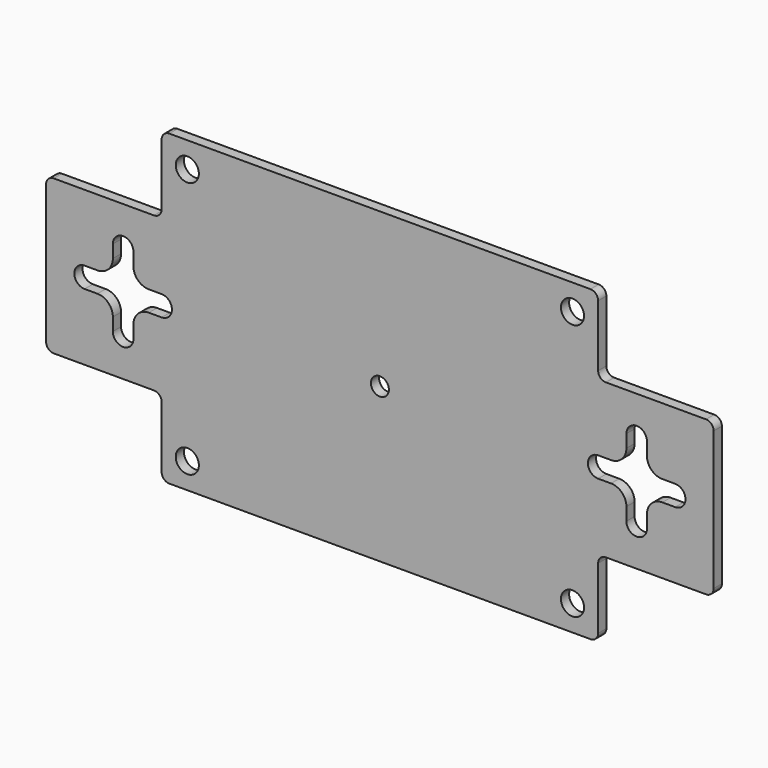
from build123d import *

# Parameters (mm, degrees)
F0_W     = 85
F0_H     = 15
F0_R     = 2.25
F0_R_2   = 1.75
F1_DEPTH = 2
F2_R     = 1.5
F3_R     = 3


# Not quite as in the source:
# - a feature names something its author has since deleted; it is built from what else it names


with BuildPart() as f1:
    # F0 (on Front) → F1 (new body)
    with BuildSketch(Plane.XZ):
        with Locations((0, 22.5)):
            Rectangle(F0_W, F0_H)
        with Locations((-37.5, 25)):
            Circle(F0_R, mode=Mode.SUBTRACT)
        with Locations((37.5, 25)):
            Circle(F0_R, mode=Mode.SUBTRACT)
        with Locations((0, -22.5)):
            Rectangle(F0_W, F0_H)
        with Locations((-37.5, -25)):
            Circle(F0_R, mode=Mode.SUBTRACT)
        with Locations((37.5, -25)):
            Circle(F0_R, mode=Mode.SUBTRACT)
        with BuildLine():
            Line((-42.5, -2), (-42.5, -15))
            Line((-42.5, -15), (42.5, -15))
            Line((42.5, -15), (42.5, -2))
            ThreePointArc((42.5, -2), (40.5, 0), (42.5, 2))
            Line((42.5, 2), (42.5, 15))
            Line((42.5, 15), (-42.5, 15))
            Line((-42.5, 15), (-42.5, 2))
            ThreePointArc((-42.5, 2), (-40.5, 0), (-42.5, -2))
        make_face()
        Circle(F0_R_2, mode=Mode.SUBTRACT)
        with BuildLine():
            Line((-65, -15), (-42.5, -15))
            Line((-42.5, -15), (-42.5, -2))
            Line((-42.5, -2), (-48, -2))
            Line((-48, -2), (-48, -7.5))
            ThreePointArc((-48, -7.5), (-50, -9.5), (-52, -7.5))
            Line((-52, -7.5), (-52, -2))
            Line((-52, -2), (-57.5, -2))
            ThreePointArc((-57.5, -2), (-59.5, 0), (-57.5, 2))
            Line((-57.5, 2), (-52, 2))
            Line((-52, 2), (-52, 7.5))
            ThreePointArc((-52, 7.5), (-50, 9.5), (-48, 7.5))
            Line((-48, 7.5), (-48, 2))
            Line((-48, 2), (-42.5, 2))
            Line((-42.5, 2), (-42.5, 15))
            Line((-42.5, 15), (-65, 15))
            Line((-65, 15), (-65, -15))
        make_face()
        with BuildLine():
            Line((42.5, -2), (42.5, -15))
            Line((42.5, -15), (65, -15))
            Line((65, -15), (65, 15))
            Line((65, 15), (42.5, 15))
            Line((42.5, 15), (42.5, 2))
            Line((42.5, 2), (48, 2))
            Line((48, 2), (48, 7.5))
            ThreePointArc((48, 7.5), (50, 9.5), (52, 7.5))
            Line((52, 7.5), (52, 2))
            Line((52, 2), (57.5, 2))
            ThreePointArc((57.5, 2), (59.5, 0), (57.5, -2))
            Line((57.5, -2), (52, -2))
            Line((52, -2), (52, -7.5))
            ThreePointArc((52, -7.5), (50, -9.5), (48, -7.5))
            Line((48, -7.5), (48, -2))
            Line((48, -2), (42.5, -2))
        make_face()
    extrude(amount=-F1_DEPTH)

    # F2
    f2_edges = [f1.edges().sort_by_distance(p)[0] for p in [
        (-42.5, 1, 30),
        (42.5, 1, 30),
        (42.5, 1, -30),
        (-42.5, 1, -30),
        (-42.5, 1, 15),
        (-65, 1, 15),
        (-65, 1, -15),
        (-42.5, 1, -15),
        (42.5, 1, 15),
        (65, 1, 15),
        (42.5, 1, -15),
        (65, 1, -15),
    ]]
    fillet(f2_edges, radius=F2_R)

    # F3
    f3_edges = [f1.edges().sort_by_distance(p)[0] for p in [
        (48, 1, 2),
        (52, 1, 2),
        (48, 1, -2),
        (52, 1, -2),
        (-48, 1, 2),
        (-52, 1, 2),
        (-48, 1, -2),
        (-52, 1, -2),
    ]]
    fillet(f3_edges, radius=F3_R)


solid = f1.part
